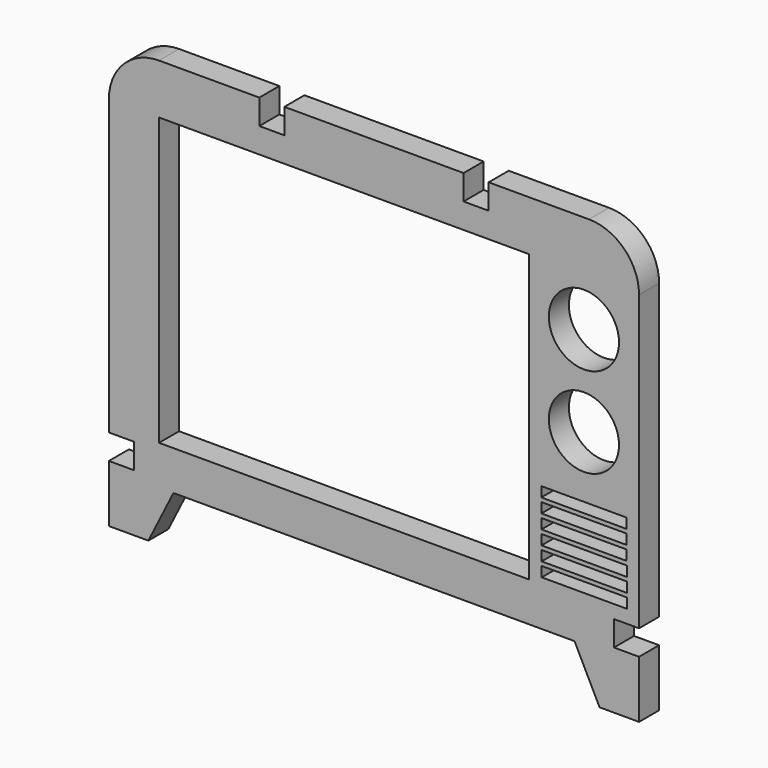
from build123d import *

# Parameters (mm, degrees)
F1_W     = 21.59
F1_H     = 2.54
F1_R     = 8.89
F2_DEPTH = 6.35


# Not quite as in the source:
# - a variable given as a bare number and used for a length is read in inches; the dataset says mm whatever the document's units were


with BuildPart() as f2:
    # F1 (on Front) → F2 (new body)
    with BuildSketch(Plane.XZ):
        with BuildLine():
            Line((-50.8, 0), (0, 0))
            Line((0, 0), (50.8, 0))
            Line((50.8, 0), (57.15, -12.7))
            Line((57.15, -12.7), (67.15, -12.7))
            Line((67.15, -12.7), (67.15, 1.825))
            Line((67.15, 1.825), (60.8, 1.825))
            Line((60.8, 1.825), (60.8, 8.175))
            Line((60.8, 8.175), (67.15, 8.175))
            Line((67.15, 8.175), (67.15, 82.55))
            ThreePointArc((67.15, 82.55), (63.4302561211, 91.5302561211), (54.45, 95.25))
            Line((54.45, 95.25), (48.1170043349, 95.25))
            Line((48.1170043349, 95.25), (29.05, 95.25))
            Line((29.05, 95.25), (29.05, 88.9))
            Line((29.05, 88.9), (22.7, 88.9))
            Line((22.7, 88.9), (22.7, 95.25))
            Line((22.7, 95.25), (0, 95.25))
            Line((0, 95.25), (-22.7, 95.25))
            Line((-22.7, 95.25), (-22.7, 88.9))
            Line((-22.7, 88.9), (-29.05, 88.9))
            Line((-29.05, 88.9), (-29.05, 95.25))
            Line((-29.05, 95.25), (-48.1170043349, 95.25))
            Line((-48.1170043349, 95.25), (-54.45, 95.25))
            ThreePointArc((-54.45, 95.25), (-63.4302561211, 91.5302561211), (-67.15, 82.55))
            Line((-67.15, 82.55), (-67.15, 70.6480368972))
            Line((-67.15, 70.6480368972), (-67.15, 8.175))
            Line((-67.15, 8.175), (-60.8, 8.175))
            Line((-60.8, 8.175), (-60.8, 1.825))
            Line((-60.8, 1.825), (-67.15, 1.825))
            Line((-67.15, 1.825), (-67.15, -12.7))
            Line((-67.15, -12.7), (-57.15, -12.7))
            Line((-57.15, -12.7), (-50.8, 0))
        make_face()
        with Locations((53.2934233144, 12.7932670589)):
            Rectangle(F1_W, F1_H, mode=Mode.SUBTRACT)
        with Locations((53.2707386515, 16.3491947024)):
            Rectangle(F1_W, F1_H, mode=Mode.SUBTRACT)
        with Locations((53.2480539886, 19.9051223459)):
            Rectangle(F1_W, F1_H, mode=Mode.SUBTRACT)
        with Locations((53.2253693257, 23.4610499895)):
            Rectangle(F1_W, F1_H, mode=Mode.SUBTRACT)
        with Locations((53.2026846629, 27.016977633)):
            Rectangle(F1_W, F1_H, mode=Mode.SUBTRACT)
        with Locations((53.18, 30.5729052765)):
            Rectangle(F1_W, F1_H, mode=Mode.SUBTRACT)
        Polygon((-54.45, 10), (-54.45, 82.55), (0, 82.55), (39.21, 82.55), (39.21, 10), (0, 10), align=None, mode=Mode.SUBTRACT)
        with Locations((53.18, 47.4004052765)):
            Circle(F1_R, mode=Mode.SUBTRACT)
        with Locations((53.18, 70.2604052765)):
            Circle(F1_R, mode=Mode.SUBTRACT)
    extrude(amount=F2_DEPTH)


solid = f2.part
